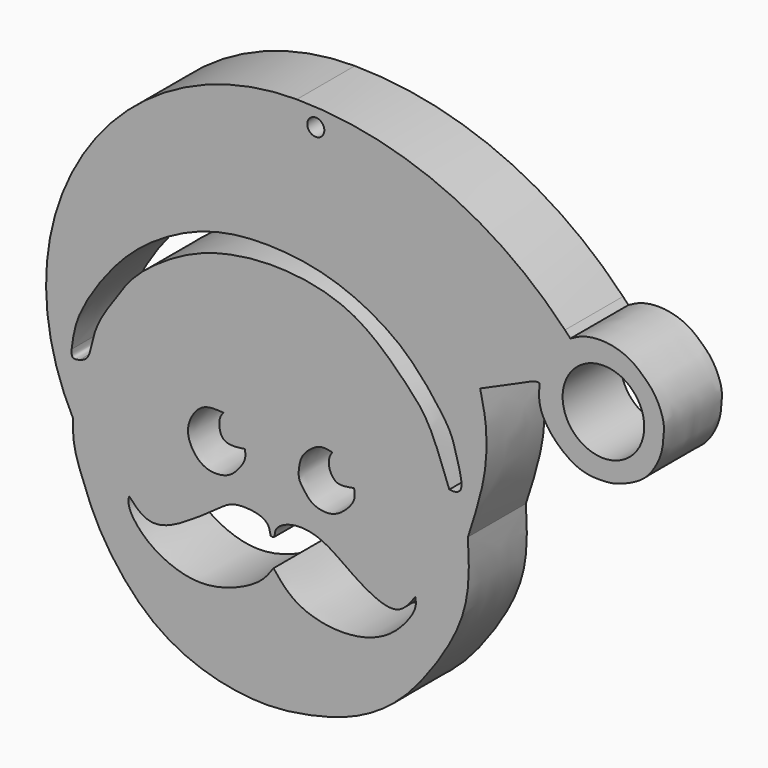
from build123d import *

# Parameters (mm, degrees)
F0_R     = 0.5893357482
F0_R_2   = 2.8141081842
F1_DEPTH = 5


# Not quite as in the source:
# - a feature names something its author has since deleted; it is built from what else it names


with BuildPart() as f1:
    # F0 (on Front) → F1 (new body)
    with BuildSketch(Plane.XZ):
        with BuildLine():
            add(Edge.make_bspline(
                [(19.1289670765, 16.4164025337), (19.2540542533, 16.2852648646), (19.3791414301, 16.1541271955), (19.5042286068, 16.0229895264)],
                knots=[0, 0, 0, 0, 0.5436865001, 0.5436865001, 0.5436865001, 0.5436865001], degree=3))
            ThreePointArc((19.1289670765, 16.4164025337), (10.7011596535, 22.2980895198), (0.6417595432, 24.4030002505))
            ThreePointArc((0.6417595432, 24.4030002505), (-9.1569529923, 21.4132843748), (-15.5417332426, 13.4015586227))
            ThreePointArc((-15.5417332426, 13.4015586227), (-16.6188020545, 6.6173603775), (-14.7759877145, 0))
            add(Edge.make_bspline(
                [(12.4396234751, 1.6734787496), (12.4928817934, 0.6318597564), (12.6013381428, -1.4893148701), (11.7071630604, -4.680326801), (8.9192131429, -8.6946605769), (6.7897968532, -10.6024037966), (4.4011204199, -11.9762510792), (1.2183804488, -12.8206077461), (-1.8401849358, -13.1689252028), (-5.8392255545, -12.550705577), (-9.8441803584, -10.5150355339), (-12.8478780093, -6.6197758149), (-13.9660340579, -3.9188799674), (-14.8148420498, -1.6333036058), (-14.7880703609, -0.5079132017), (-14.7759877145, 0)],
                knots=[0, 0, 0, 0, 0.0748995289, 0.1525269617, 0.2461251435, 0.3183095626, 0.3878882602, 0.4646057524, 0.5393839055, 0.6238972099, 0.7143196234, 0.8077384253, 0.8811819485, 0.9463748254, 1, 1, 1, 1], degree=3))
            add(Edge.make_bspline(
                [(13.2837789133, 10.9677538276), (13.4383964182, 10.3008942014), (13.7783001215, 8.8349019993), (13.7408778209, 5.7032512612), (12.8974252548, 3.0912162071), (12.4396234751, 1.6734787496)],
                knots=[0, 0, 0, 0, 0.2761742468, 0.6071282117, 1, 1, 1, 1], degree=3))
            add(Edge.make_bspline(
                [(17.3889175057, 12.6349059865), (17.3071399145, 12.6441407774), (17.0736526382, 12.6705074893), (16.1292568481, 12.2278389528), (14.4071616214, 11.4652301296), (13.2837789133, 10.9677538276)],
                knots=[0, 0, 0, 0, 0.157827672, 0.4506216522, 1, 1, 1, 1], degree=3))
            add(Edge.make_bspline(
                [(19.5042286068, 16.0229895264), (19.7618793826, 16.1664952467), (20.3465515008, 16.4921445415), (21.8525723701, 16.715028554), (23.5277898319, 16.2521187136), (24.4768736198, 15.4383952236), (25.4020094443, 14.5629290823), (25.9802324209, 13.1241412335), (25.9462940214, 12.3019745652), (25.8458566723, 11.0346500909), (25.1979175637, 9.8112660026), (24.4132495686, 8.9256962736), (22.7501028456, 8.1918078917), (21.8413916583, 8.1018117524), (20.5467040461, 8.1022445142), (19.3286692564, 8.6742125966), (18.0708096962, 9.787323101), (17.2636977855, 11.2527872126), (17.3484555674, 12.1883053668), (17.3889175057, 12.6349059865)],
                knots=[0, 0, 0, 0, 0.0494571537, 0.1122302804, 0.179235963, 0.2359304627, 0.293985366, 0.3563297379, 0.4029155974, 0.4598332953, 0.5195211699, 0.5757923961, 0.6434381262, 0.6932360544, 0.7498990502, 0.8090789477, 0.8754473822, 0.9405406768, 1, 1, 1, 1], degree=3))
        make_face()
        with BuildLine():
            add(Edge.make_bspline(
                [(-0.9638228221, -4.5772111043), (-1.2495453437, -4.98397497), (-1.9397858162, -5.9666237341), (-5.0833422127, -7.2888256569), (-7.6239923855, -6.970166186), (-9.7782624226, -5.8414669289), (-11.0319235293, -4.2502833325), (-10.9589660125, -3.6579344108), (-10.9308827668, -3.4299239051)],
                knots=[0, 0, 0, 0, 0.150570497, 0.3637439933, 0.5525204428, 0.7367146178, 0.8986546089, 1, 1, 1, 1], degree=3))
            add(Edge.make_bspline(
                [(-10.9308827668, -3.4299239051), (-10.6222594198, -3.7663698968), (-9.995416145, -4.4497236006), (-8.3092593265, -4.7256884897), (-6.0143972146, -3.0784152173), (-4.5311697759, -2.0137408283)],
                knots=[0, 0, 0, 0, 0.2554033012, 0.5187483166, 1, 1, 1, 1], degree=3))
            add(Edge.make_bspline(
                [(-4.5311697759, -2.0137408283), (-4.2967863236, -1.8512654848), (-3.7584325512, -1.4780769629), (-2.2016565057, -1.5112649146), (-1.3055335554, -1.9215931489), (-1.2071093018, -2.436066182), (-1.161012915, -2.6770164259)],
                knots=[0, 0, 0, 0, 0.2393599669, 0.5497842955, 0.7891442761, 1, 1, 1, 1], degree=3))
            add(Edge.make_bspline(
                [(-1.161012915, -2.6770164259), (-1.0675721443, -2.7005474096), (-0.8372609343, -2.7585461751), (-0.9492487174, -2.0288737658), (0.4080149613, -1.3283155357), (2.3464888317, -1.621081544), (4.0763433279, -2.9058644961), (5.9482987592, -4.1502345757), (7.7352715038, -4.5982184912), (8.4464108727, -3.6318248378), (8.8060470298, -3.1431019306)],
                knots=[0, 0, 0, 0, 0.0521840457, 0.1286223414, 0.2530633649, 0.402631775, 0.5616659676, 0.7255916889, 0.8612267092, 1, 1, 1, 1], degree=3))
            add(Edge.make_bspline(
                [(8.8060470298, -3.1431019306), (8.8456422518, -3.3399706171), (8.9564316104, -3.8908187855), (7.5879277489, -5.7614752214), (5.5558981074, -6.8324022566), (2.9612847768, -7.0397264538), (0.3988413132, -6.2657680799), (-0.5249223295, -5.1210784221), (-0.9638228221, -4.5772111043)],
                knots=[0, 0, 0, 0, 0.0962923404, 0.2694306559, 0.450097876, 0.6390207725, 0.8284908028, 1, 1, 1, 1], degree=3))
        make_face(mode=Mode.SUBTRACT)
        with BuildLine():
            add(Edge.make_bspline(
                [(-2.9357231688, 2.0196919795), (-2.905913156, 1.8219933905), (-2.8383829968, 1.3741365811), (-3.4465600278, 0.5262452687), (-4.1655653648, -0.120855501), (-5.7103713292, -0.2026802663), (-6.7309797319, 0.9099976684), (-7.0061932668, 2.1862913586), (-6.2395765771, 3.4597187073), (-5.4003089146, 3.8083914533), (-4.7553924488, 3.7636437948), (-4.4236117974, 3.7406231277)],
                knots=[0, 0, 0, 0, 0.0841361117, 0.190597873, 0.2961541438, 0.4226355898, 0.5496652109, 0.6692874203, 0.7949418536, 0.8945067633, 1, 1, 1, 1], degree=3))
            add(Edge.make_bspline(
                [(-4.4236117974, 3.7406231277), (-4.5056994985, 3.6311775702), (-4.6856300133, 3.3912805423), (-4.7331747586, 2.7869335369), (-4.5330680055, 2.1037799557), (-3.8642846788, 1.8845814454), (-3.2666277247, 1.9715436438), (-2.9357231688, 2.0196919795)],
                knots=[0, 0, 0, 0, 0.162135371, 0.3553894238, 0.5579393274, 0.755244393, 1, 1, 1, 1], degree=3))
        make_face(mode=Mode.SUBTRACT)
        with BuildLine():
            add(Edge.make_bspline(
                [(4.5933509246, 2.0913975313), (4.6290595615, 1.8687515173), (4.7099375499, 1.3644712285), (3.9703271967, 0.4612921887), (2.9585555451, -0.1564583704), (1.6091484533, 0.1301345246), (1.0941784969, 0.9499665974), (0.692167638, 1.4411492785), (0.8399801779, 2.4957761744), (1.0957848097, 3.09869217), (2.1462008326, 3.9900826386), (2.7902208047, 3.8439424494), (3.087536199, 3.77647602)],
                knots=[0, 0, 0, 0, 0.085123855, 0.1928005869, 0.3042570232, 0.4194299636, 0.5180358454, 0.5985549479, 0.7001682351, 0.786305469, 0.9013467338, 1, 1, 1, 1], degree=3))
            add(Edge.make_bspline(
                [(3.087536199, 3.77647602), (3.0200768522, 3.6776153169), (2.8737280477, 3.4631432477), (2.8154727911, 2.9400659536), (2.9879999799, 2.4440641375), (3.2955409371, 2.0408035287), (3.7888857188, 1.9448402237), (4.3002273289, 2.0379963343), (4.5933509246, 2.0913975313)],
                knots=[0, 0, 0, 0, 0.1406080133, 0.3050402295, 0.4730840461, 0.6318375704, 0.7889530345, 1, 1, 1, 1], degree=3))
        make_face(mode=Mode.SUBTRACT)
        with BuildLine():
            add(Edge.make_bspline(
                [(-14.3466116861, 3.710525576), (-14.1478705114, 3.7762222556), (-13.6745324002, 3.9326907995), (-13.4879557887, 5.2145391348), (-12.9717119675, 6.6650458536), (-11.8674148369, 8.2302122455), (-10.9428783287, 9.6665498669), (-9.2613111972, 11.1914063485), (-6.444363323, 12.8936842722), (-3.3523104294, 13.7071314962), (0.0640277441, 13.9091252706), (4.8179887271, 13.0307519837), (8.4179944287, 9.3812096461), (9.8099017521, 7.794368107), (10.665831875, 5.4737442158), (11.157209985, 4.1415048763)],
                knots=[0, 0, 0, 0, 0.038122513, 0.090795671, 0.1523067408, 0.2192700475, 0.2825352378, 0.3551625311, 0.4433728329, 0.5299427508, 0.619351732, 0.7260710873, 0.8337824409, 0.904576708, 1, 1, 1, 1], degree=3))
            add(Edge.make_bspline(
                [(-14.8789975792, 4.1922079399), (-14.8867442966, 3.9908164209), (-14.9019757045, 3.5948452965), (-14.5295976788, 3.6724102677), (-14.3466116861, 3.710525576)],
                knots=[0, 0, 0, 0, 0.5086015283, 1, 1, 1, 1], degree=3))
            add(Edge.make_bspline(
                [(9.6361069009, 9.8963426426), (9.1068635196, 10.5017354525), (7.9817398995, 11.788745879), (5.2711923509, 13.5004449308), (2.0320658811, 14.7039090453), (-2.1722151929, 15.0853302821), (-6.1097101471, 14.4568832336), (-10.059706776, 12.218551294), (-12.6038380306, 9.5329342087), (-14.62167668, 6.30996414), (-14.8019726615, 4.8261245689), (-14.8789975792, 4.1922079399)],
                knots=[0, 0, 0, 0, 0.0945227027, 0.2009467273, 0.3129220147, 0.4353387198, 0.5554223079, 0.6815147731, 0.7986672444, 0.9139878837, 1, 1, 1, 1], degree=3))
            add(Edge.make_bspline(
                [(11.157209985, 4.1415048763), (11.299627538, 4.1263929616), (11.5959360634, 4.0949516886), (12.234608816, 4.4318395759), (11.5571861475, 6.5950141493), (11.2783815639, 7.8017710806), (10.2390366988, 9.1273606709), (9.6361069009, 9.8963426426)],
                knots=[0, 0, 0, 0, 0.1176356321, 0.2447482067, 0.5003038359, 0.7101234467, 1, 1, 1, 1], degree=3))
        make_face(mode=Mode.SUBTRACT)
        with Locations((1.9503255608, 23.1382679194)):
            Circle(F0_R, mode=Mode.SUBTRACT)
        with Locations((21.7817405815, 12.3112803198)):
            Circle(F0_R_2, mode=Mode.SUBTRACT)
    extrude(amount=F1_DEPTH)


solid = f1.part
